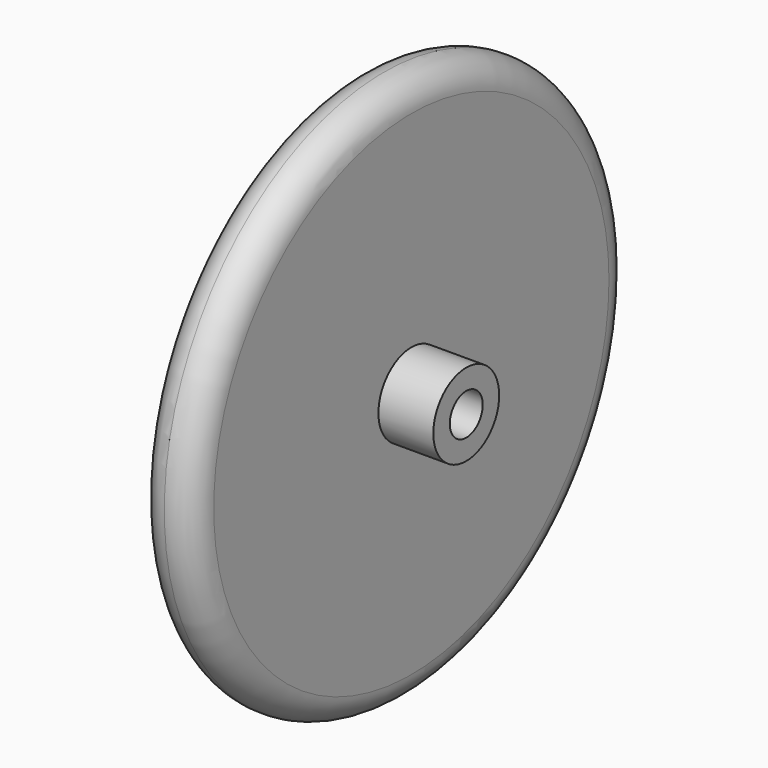
from build123d import *

# Parameters (mm, degrees)
F0_R     = 10
F1_DEPTH = 2
F2_R     = 1.5
F2_R_2   = 0.75
F3_DEPTH = 2
F4_R     = 0.99999


# Not quite as in the source:
# - a fillet or chamfer is up to 0.001 mm smaller than in the source, because OpenCascade refuses the exact size


with BuildPart() as f1:
    # F0 (on Right) → F1 (new body)
    with BuildSketch(Plane.YZ):
        with Locations((36.0975265503, 19.3211734295)):
            Circle(F0_R)
    extrude(amount=F1_DEPTH)

    # F2 (on face) → F3 (join)
    with BuildSketch(Plane.YZ.offset(2)):
        with Locations((36.0975265503, 19.3211734295)):
            Circle(F2_R)
        with Locations((36.0975265503, 19.3211734295)):
            Circle(F2_R_2, mode=Mode.SUBTRACT)
    extrude(amount=F3_DEPTH)

    # F4 (radius 1 in the source; OpenCascade refuses exactly that, so slightly less here)
    f4_edges = [f1.edges().sort_by_distance(p)[0] for p in [
        (2, 26.097527, 19.321173),
        (0, 26.097527, 19.321173),
    ]]
    fillet(f4_edges, radius=F4_R)


solid = f1.part
